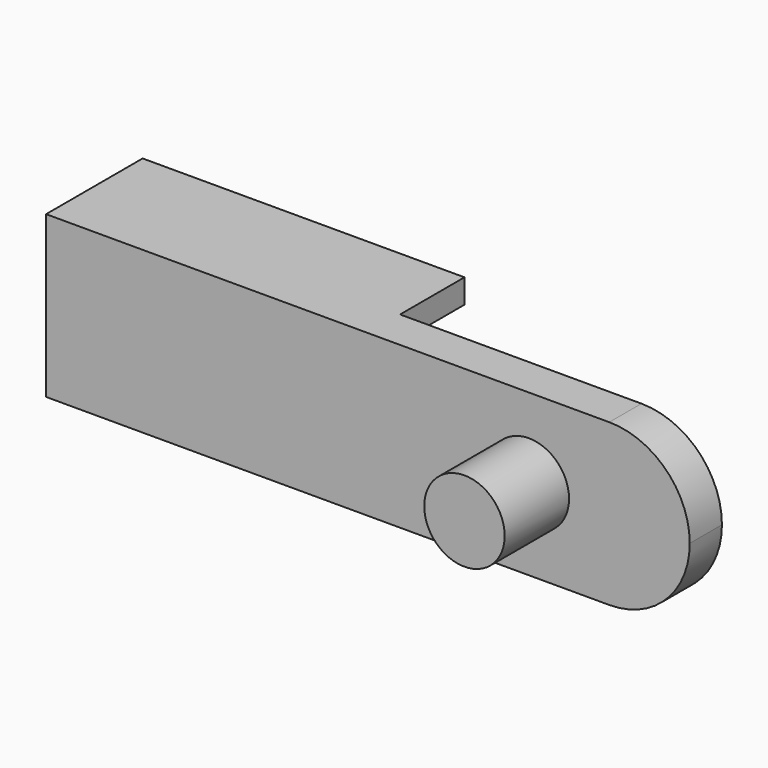
from build123d import *

# Parameters (mm, degrees)
F0_W     = 50.8
F0_H     = 12.7
F1_DEPTH = 3.175
F2_R     = 3.175
F3_DEPTH = 6.35
F5_DEPTH = 6.35
F6_R     = 3.175
F7_R     = 6.34999


# Not quite as in the source:
# - a fillet or chamfer is up to 0.001 mm smaller than in the source, because OpenCascade refuses the exact size


with BuildPart() as f1:
    # F0 (on Front) → F1 (new body)
    with BuildSketch(Plane.XZ):
        with Locations((25.4, 6.35)):
            Rectangle(F0_W, F0_H)
    extrude(amount=F1_DEPTH)

    # F2 (on face) → F3 (join)
    with BuildSketch(Plane.XZ.offset(3.175)):
        with Locations((38.1, 6.35)):
            Circle(F2_R)
    extrude(amount=F3_DEPTH)

    # F4 (on face) → F5 (join)
    with BuildSketch(Plane(origin=(0, 0, 0), x_dir=(-1, 0, 0), z_dir=(0, 1, 0))):
        Polygon((0, 0), (0, 12.7), (-25.4, 12.7), (-25.4, 10.795), (-1.905, 10.795), (-1.905, 1.905), (-25.4, 1.905), (-25.4, 0), align=None)
    extrude(amount=F5_DEPTH)

    # F6
    f6_edges = [f1.edges().sort_by_distance(p)[0] for p in [
        (1.905, 3.175, 10.795),
        (1.905, 3.175, 1.905),
    ]]
    fillet(f6_edges, radius=F6_R)

    # F7 (radius 6.35 in the source; OpenCascade refuses exactly that, so slightly less here)
    f7_edges = [f1.edges().sort_by_distance(p)[0] for p in [
        (50.8, -1.5875, 12.7),
        (50.8, -1.5875, 0),
    ]]
    fillet(f7_edges, radius=F7_R)


solid = f1.part
